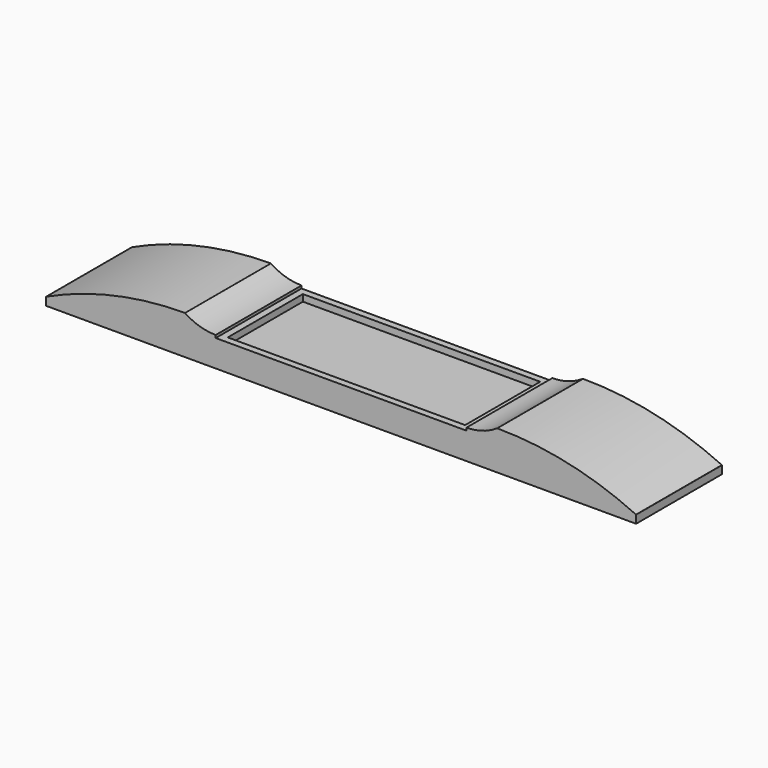
from build123d import *

# Parameters (mm, degrees)
F1_DEPTH = 80
F3_W     = 177
F3_H     = 70
F4_DEPTH = 5


# Not quite as in the source:
# - ends of sketch curves that miss each other by under 0.0002 mm in the source are joined


with BuildPart() as f1:
    # F0 (on Front) → F1 (new body)
    with BuildSketch(Plane.XZ):
        with BuildLine():
            Line((-220, 0), (0, 0))
            Line((0, 0), (220, 0))
            Line((220, 0), (220, 5.872634))
            ThreePointArc((220, 5.872634), (219.9686827703, 5.9800868873), (219.8845387701, 6.0538885071))
            ThreePointArc((219.8845387701, 6.0538885071), (169.4297421053, 23.1880267358), (116.462901, 28.9999923785))
            ThreePointArc((116.462901, 28.9999923785), (116.4045566452, 28.9913078859), (116.3512831377, 28.9659817952))
            ThreePointArc((116.3512831377, 28.9659817952), (105.4447272771, 23.7801763601), (93.5, 22))
            Line((93.5, 22), (93.5, 20))
            Line((93.5, 20), (0, 20))
            Line((0, 20), (-93.5, 20))
            Line((-93.5, 20), (-93.5, 22))
            ThreePointArc((-93.5, 22), (-105.4447272771, 23.7801763601), (-116.351282957, 28.965982064))
            ThreePointArc((-116.351282957, 28.965982064), (-116.4045566452, 28.9913078859), (-116.462901, 28.9999919938))
            ThreePointArc((-116.462901, 28.9999919938), (-169.4297421053, 23.1880267358), (-219.8845388425, 6.0538886623))
            ThreePointArc((-219.8845388425, 6.0538886623), (-219.9686827703, 5.9800868873), (-220, 5.872634))
            Line((-220, 5.872634), (-220, 0))
        make_face()
    extrude(amount=F1_DEPTH)

    # F3 (on face) → F4 (cut)
    with BuildSketch(Plane.XY.offset(20)):
        with Locations((0, -40)):
            Rectangle(F3_W, F3_H)
    extrude(amount=-F4_DEPTH, mode=Mode.SUBTRACT)


solid = f1.part
